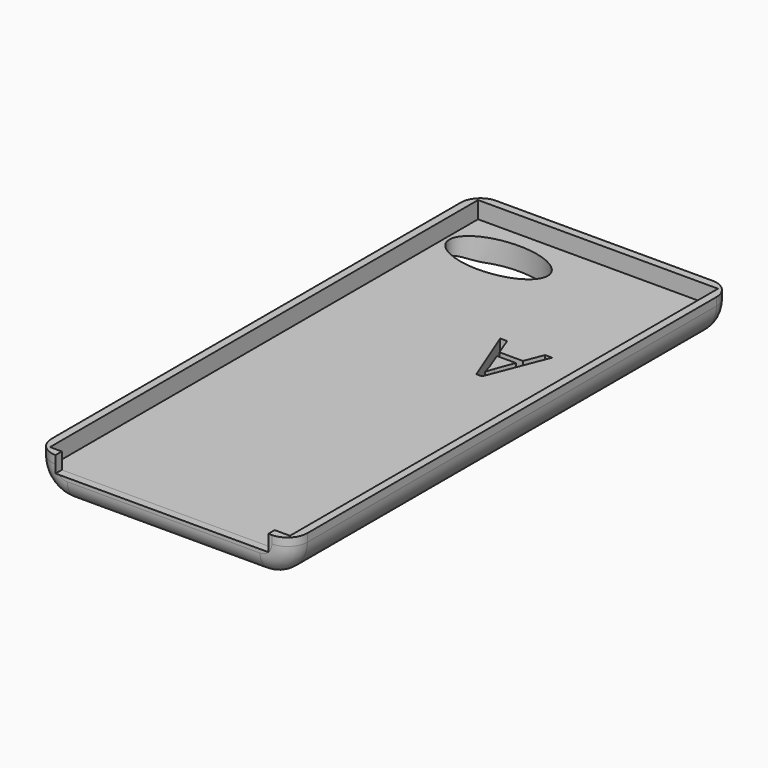
from build123d import *

# Parameters (mm, degrees)
F0_W          = 65
F0_H          = 140
F1_DEPTH      = 10
F2_R          = 8
F3_W          = 61.0000006855
F3_H          = 136.0000006855
F4_DEPTH      = 6.5
F5_DEPTH      = 4.3
F7_DEPTH      = 10.001
F8_R          = 5
F9_W          = 54.1213203436
F9_H          = 4.1213203436
F10_DEPTH     = 1.9999996573
F11_TEXT_SIZE = 20.8520679735
F12_DEPTH     = 5.7


# Not quite as in the source:
# - Text() gives the source's letters only with a copy of the font that has no kerning and outlines rounded to 1/6400 em; it was checked with that copy


with BuildPart() as f1:
    # F0 (on Top) → F1 (new body)
    with BuildSketch(Plane.XY):
        Rectangle(F0_W, F0_H)
    extrude(amount=F1_DEPTH)

    # F2
    f2_edges = [f1.edges().sort_by_distance(p)[0] for p in [
        (32.5, 0, 0),
        (-32.5, 0, 0),
    ]]
    fillet(f2_edges, radius=F2_R)

    # F3 (on face) → F4 (join)
    with BuildSketch(Plane.XY.offset(10)):
        Rectangle(F3_W, F3_H)
    extrude(amount=-F4_DEPTH)

    # F3 (on face) → F5 (cut)
    with BuildSketch(Plane.XY.offset(10)):
        Rectangle(F3_W, F3_H)
    extrude(amount=-F5_DEPTH, mode=Mode.SUBTRACT)

    # F6 (on face) → F7 (cut, through all)
    with BuildSketch(Plane.XY.offset(10)):
        with BuildLine():
            add(Edge.make_bspline(
                [(-4.5, 57.6461367309), (-4.5, 68.9044669801), (-23.25, 63.2753018555), (-42, 57.6461367309), (-23.25, 52.0169716063), (-4.5, 46.3878064817), (-4.5, 57.6461367309)],
                knots=[0, 0, 0, 2.0943951024, 2.0943951024, 4.1887902048, 4.1887902048, 6.2831853072, 6.2831853072, 6.2831853072], degree=2, weights=[1, 0.5, 1, 0.5, 1, 0.5, 1]))
        make_face()
    extrude(amount=-F7_DEPTH, mode=Mode.SUBTRACT)

    # F8
    f8_edges = [f1.edges().sort_by_distance(p)[0] for p in [
        (0, 70, 0),
        (0, -70, 0),
    ]]
    fillet(f8_edges, radius=F8_R)

    # F9 (on face) → F10 (cut, through all)
    with BuildSketch(Plane.XZ.offset(70)):
        with Locations((-0.4393398282, 7.9393398282)):
            Rectangle(F9_W, F9_H)
    extrude(amount=-F10_DEPTH, mode=Mode.SUBTRACT)

    # F11 (on face) → F12 (cut, through all)
    with BuildSketch(Plane(origin=(0, 0, 0), x_dir=(1, 0, 0), z_dir=(0, 0, -1))):
        with Locations((4.9572843127, -30.7351639494)):
            Text('A', F11_TEXT_SIZE, font='Open Sans', text_align=(TextAlign.LEFT, TextAlign.BOTTOM))
    extrude(amount=-F12_DEPTH, mode=Mode.SUBTRACT)


solid = f1.part
